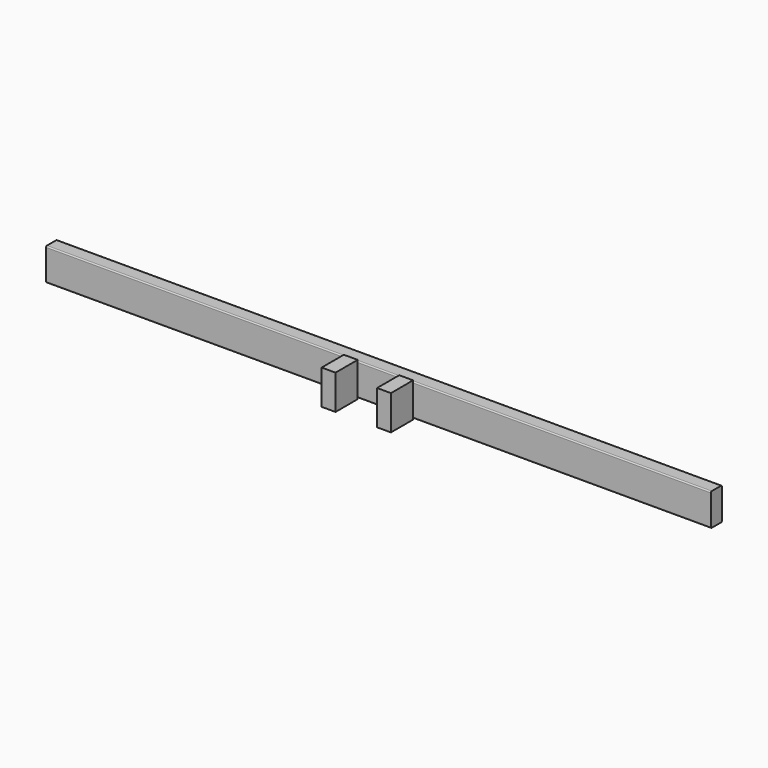
from build123d import *

# Parameters (mm, degrees)
F0_W     = 38.1
F0_H     = 88.9
F1_DEPTH = 914.4
F2_R     = 3.175
F4_W     = 38.1
F4_H     = 95.25
F5_DEPTH = 76.2


with BuildPart() as f1:
    # F0 (on Right) → F1 (new body, symmetric)
    with BuildSketch(Plane.YZ):
        Rectangle(F0_W, F0_H)
    extrude(amount=F1_DEPTH, both=True)

    # F2
    f2_edges = [f1.edges().sort_by_distance(p)[0] for p in [
        (0, -19.05, 44.45),
        (0, 19.05, 44.45),
        (0, -19.05, -44.45),
        (0, 19.05, -44.45),
    ]]
    fillet(f2_edges, radius=F2_R)

    # F4 (on face) → F5 (join)
    with BuildSketch(Plane.XZ.offset(19.05)):
        with Locations((76.2, 0)):
            Rectangle(F4_W, F4_H)
    extrude(amount=F5_DEPTH)

    # F6: F1 across plane


with BuildPart() as f1_1:
    add(f1.part)
    add(f1.part.mirror(Plane.YZ))


solid = f1_1.part
